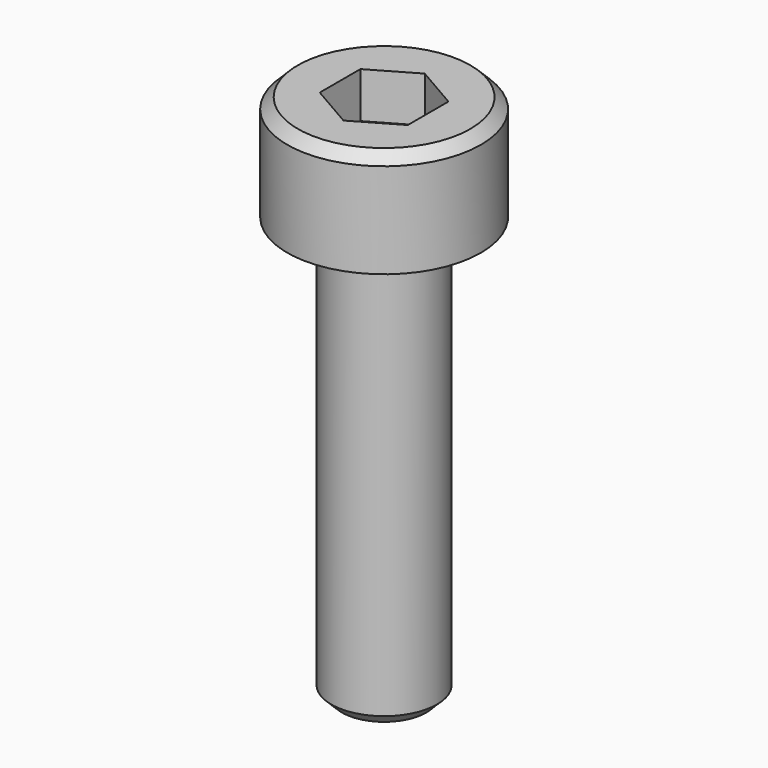
from build123d import *

# Parameters (mm, degrees)
F2_R      = 1.5
F3_DEPTH  = 12
F2_R_2    = 2.75
F3_FACE_R = 1.5
F4_DEPTH  = 3
F5_SIZE   = 0.3
F7_DEPTH  = 1.3


with BuildPart() as f3:
    # F2 (on Top) → F3 (new body)
    with BuildSketch(Plane.XY):
        Circle(F2_R)
    extrude(amount=-F3_DEPTH)

    # F2 (on Top) + F3_face (on face) → F4 (join)
    with BuildSketch(Plane.XY):
        Circle(F2_R_2)
        Circle(F2_R, mode=Mode.SUBTRACT)
    with BuildSketch(Plane.XY):
        Circle(F3_FACE_R)
    extrude(amount=F4_DEPTH)

    # F5
    f5_edges = [f3.edges().sort_by_distance(p)[0] for p in [
        (-1.5, 0, -12),
        (-2.75, 0, 3),
    ]]
    chamfer(f5_edges, length=F5_SIZE)

    # F6 (on face) → F7 (cut)
    with BuildSketch(Plane.XY.offset(3)):
        Polygon((1.25, -0.7216878365), (1.25, 0.7216878365), (0, 1.443375673), (-1.25, 0.7216878365), (-1.25, -0.7216878365), (0, -1.443375673), align=None)
    extrude(amount=-F7_DEPTH, mode=Mode.SUBTRACT)


solid = f3.part
